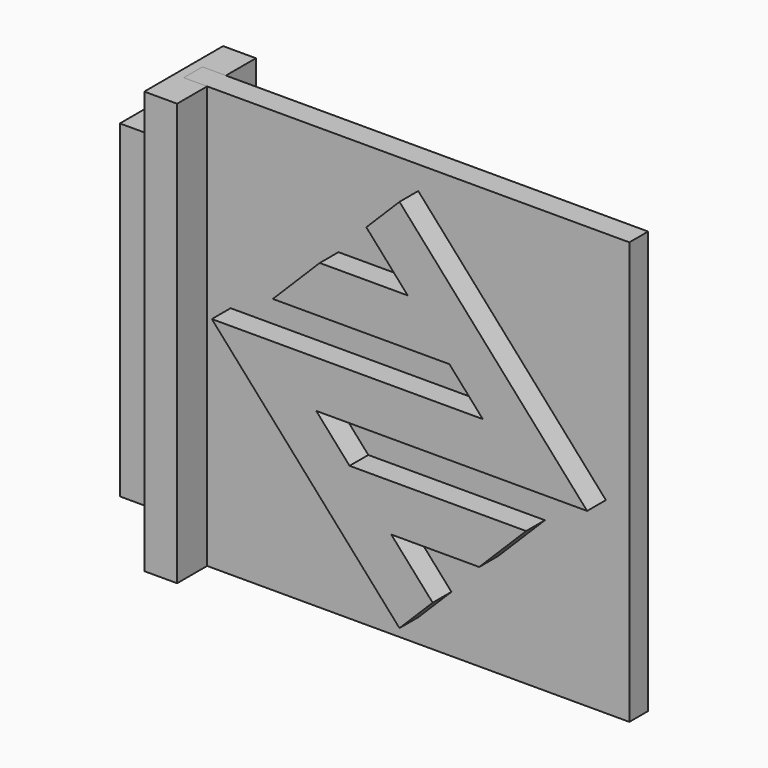
from build123d import *

# Parameters (mm, degrees)
F1_DEPTH  = 25
F2_W      = 70
F2_H      = 800
F3_DEPTH  = 80
F5_W      = 20
F5_H      = 50
F6_DEPTH  = 800
F8_DEPTH  = 50
F11_W     = 140
F11_H     = 700
F12_DEPTH = 80
F13_DEPTH = 50
F14_DEPTH = 50


with BuildPart() as f1:
    # F0 (on Front) → F1 (new body, symmetric)
    with BuildSketch(Plane.XZ):
        Polygon((450, 450), (-450, 450), (-500, 450), (-500, -450), (-450, -450), (450, -450), align=None)
    extrude(amount=F1_DEPTH, both=True)


with BuildPart() as f3:
    # F2 (on face) → F3 (new body)
    with BuildSketch(Plane.XZ.offset(25)):
        with Locations((-485, 0)):
            Rectangle(F2_W, F2_H)
    extrude(amount=F3_DEPTH)


with BuildPart() as f4_1:
    # F4: instance of F3
    add(f3.part.mirror(Plane.XZ))


with BuildPart() as f3_1:
    add(f3.part)

    add(f4_1.part)  # F6 merges F4_1
    # F5 (on face) → F6 (join, through all)
    with BuildSketch(Plane.XY.offset(400)):
        with Locations((-510, 0)):
            Rectangle(F5_W, F5_H)
    extrude(amount=-F6_DEPTH)

    # F13 (add, through all): a face of the model
    f13_faces = [f3_1.faces().sort_by_distance(p)[0] for p in [
        (-452.2135943621, 65, 400),
    ]]
    extrude(f13_faces, amount=F13_DEPTH)

    # F14 (add, through all): a face of the model
    f14_faces = [f3_1.faces().sort_by_distance(p)[0] for p in [
        (-517.7864056379, 0, -400),
    ]]
    extrude(f14_faces, amount=F14_DEPTH)


with BuildPart() as f8:
    # F7 (on face) → F8 (new body)
    with BuildSketch(Plane.XZ.offset(25)):
        Polygon((-400, 50), (0, -400), (70.7106781187, -329.2893218813), (-17.546496887, -230), (170, -230), (270, -130), (-106.4353857759, -130), (-177.546496887, -50), (400, -50), (0, 400), (-70.7106781187, 329.2893218813), (17.546496887, 230), (-170, 230), (-270, 130), (106.4353857759, 130), (177.546496887, 50), align=None)
    extrude(amount=F8_DEPTH)


with BuildPart() as f9_1:
    # F9: instance of F8
    add(f8.part.mirror(Plane.XZ))


with BuildPart() as f10_1:
    # F10: instance of F9_1
    add(f9_1.part.mirror(Plane.YZ))


with BuildPart() as f12:
    # F11 (on face) → F12 (new body)
    with BuildSketch(Plane(origin=(-520, 0, 0), x_dir=(0, -1, 0), z_dir=(-1, 0, 0))):
        Rectangle(F11_W, F11_H)
    extrude(amount=F12_DEPTH)


solid = Compound([f1.part, f3_1.part, f8.part, f9_1.part, f10_1.part, f12.part])
